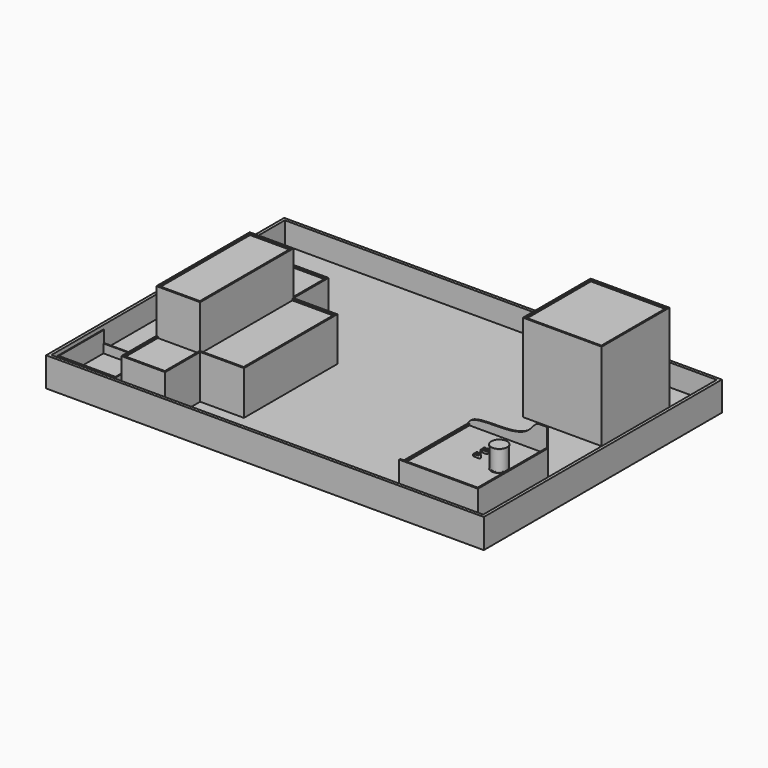
from build123d import *

# Parameters (mm, degrees)
F0_R      = 27.2
F1_DEPTH  = 2.83
F2_R      = 26.4
F3_DEPTH  = 67.36
F4_R      = 27.2
F5_DEPTH  = 2.83
F9_W      = 270
F9_H      = 300
F10_DEPTH = 72
F12_DEPTH = 15
F14_DEPTH = 5
F15_W     = 5
F15_H     = 290
F16_DEPTH = 5
F17_W     = 1500
F17_H     = 1020
F18_DEPTH = 25
F19_W     = 270
F19_H     = 290
F20_DEPTH = 300
F21_W     = 260
F21_H     = 280
F22_DEPTH = 5
F23_W     = 1500
F23_H     = 1020
F23_W_2   = 1480
F23_H_2   = 1000
F24_DEPTH = 75
F26_DEPTH = 150
F27_W     = 150
F27_H     = 400
F28_DEPTH = 150
F29_W     = 140
F29_H     = 390
F30_DEPTH = 5
F31_W     = 140
F31_H     = 145
F31_W_2   = 145
F31_H_2   = 390
F32_DEPTH = 5
F33_R     = 3
F34_DEPTH = 4
F35_R     = 3.99999
F35_2_R   = 3.99999
F36_R     = 3
F37_DEPTH = 8
F38_R     = 3
F39_DEPTH = 8
F40_R     = 3
F40_R_2   = 2.5
F41_DEPTH = 3
F42_R     = 3
F42_R_2   = 2.5
F43_DEPTH = 3
F45_DEPTH = 270.001
F46_W     = 200
F46_H     = 200
F46_W_2   = 194
F46_H_2   = 191
F47_DEPTH = 30
F49_DEPTH = 40
F50_R     = 2.5403619878
F51_DEPTH = 6
F50_R_2   = 2.6285420135
F50_R_3   = 2.461967709
F50_R_4   = 2.4586880428


# Not quite as in the source:
# - a fillet or chamfer is up to 0.001 mm smaller than in the source, because OpenCascade refuses the exact size
# - a feature names something its author has since deleted; it is built from what else it names


with BuildPart() as f1:
    # F0 (on Top) → F1 (new body)
    with BuildSketch(Plane.XY):
        Circle(F0_R)
    extrude(amount=F1_DEPTH)

    # F2 (on face) → F3 (join)
    with BuildSketch(Plane.XY.offset(2.83)):
        Circle(F2_R)
    extrude(amount=F3_DEPTH)

    # F4 (on face) → F5 (join)
    with BuildSketch(Plane.XY.offset(70.19)):
        Circle(F4_R)
    extrude(amount=F5_DEPTH)


with BuildPart() as f10:
    # F9 (on Top) → F10 (new body)
    with BuildSketch(Plane.XY):
        with Locations((-87.8, 0)):
            Rectangle(F9_W, F9_H)
    extrude(amount=-F10_DEPTH)

    # F11 (on face) → F12 (join)
    with BuildSketch(Plane.XY):
        Polygon((-222.8, -145), (-222.8, -150), (47.2, -150), (47.2, 150), (42.2, 150), (42.2, -145), align=None)
    extrude(amount=F12_DEPTH)

    # F13 (on face) → F14 (join)
    with BuildSketch(Plane(origin=(0, 150, 0), x_dir=(-1, 0, 0), z_dir=(0, 1, 0))):
        with BuildLine():
            Line((-21.3134280931, 81.3575685024), (-47.2, 81.3575685024))
            Line((-47.2, 81.3575685024), (-47.2, -72))
            Line((-47.2, -72), (222.8, -72))
            Line((222.8, -72), (222.8, 0))
            add(Edge.make_bspline(
                [(-21.3134280931, 81.3575685024), (-6.3059147253, 81.3822787863), (12.9585432644, 38.1268753575), (103.6097013063, 23.6068887567), (223.0224295336, 30.7718731823), (222.8, 0)],
                knots=[0, 0, 0, 0, 0.2487100673, 0.6151112321, 1, 1, 1, 1], degree=3))
        make_face()
    extrude(amount=-F14_DEPTH)

    # F15 (on face) → F16 (join)
    with BuildSketch(Plane.XY):
        with Locations((-220.3, 0)):
            Rectangle(F15_W, F15_H)
    extrude(amount=F16_DEPTH)

    # F17 (on face) → F18 (join)
    with BuildSketch(Plane(origin=(0, 0, -72), x_dir=(1, 0, 0), z_dir=(0, 0, -1))):
        with Locations((-602.8, -260)):
            Rectangle(F17_W, F17_H)
    extrude(amount=F18_DEPTH)

    # F19 (on face) → F20 (join)
    with BuildSketch(Plane.XY.offset(-72)):
        with Locations((-87.8, 525)):
            Rectangle(F19_W, F19_H)
    extrude(amount=F20_DEPTH)

    # F21 (on face) → F22 (cut)
    with BuildSketch(Plane.XY.offset(228)):
        with Locations((-87.8, 525)):
            Rectangle(F21_W, F21_H)
    extrude(amount=-F22_DEPTH, mode=Mode.SUBTRACT)

    # F23 (on face) → F24 (join)
    with BuildSketch(Plane.XY.offset(-72)):
        with Locations((-602.8, 260)):
            Rectangle(F23_W, F23_H)
        with Locations((-602.8, 260)):
            Rectangle(F23_W_2, F23_H_2, mode=Mode.SUBTRACT)
    extrude(amount=F24_DEPTH)

    # F25 (on face) → F26 (join)
    with BuildSketch(Plane.XY.offset(-72)):
        Polygon((-952.8, 460), (-1102.8, 460), (-1102.8, -240), (-952.8, -240), (-952.8, -90), (-802.8, -90), (-802.8, 310), (-952.8, 310), align=None)
    extrude(amount=F26_DEPTH)

    # F27 (on face) → F28 (join)
    with BuildSketch(Plane.XY.offset(78)):
        with Locations((-1027.8, 110)):
            Rectangle(F27_W, F27_H)
    extrude(amount=F28_DEPTH)

    # F29 (on face) → F30 (cut)
    with BuildSketch(Plane.XY.offset(228)):
        with Locations((-1027.8, 110)):
            Rectangle(F29_W, F29_H)
    extrude(amount=-F30_DEPTH, mode=Mode.SUBTRACT)

    # F31 (on face) → F32 (cut)
    with BuildSketch(Plane.XY.offset(78)):
        with Locations((-1027.8, 382.5)):
            Rectangle(F31_W, F31_H)
        with Locations((-880.3, 110)):
            Rectangle(F31_W_2, F31_H_2)
        with Locations((-1027.8, -162.5)):
            Rectangle(F31_W, F31_H)
    extrude(amount=-F32_DEPTH, mode=Mode.SUBTRACT)

    # F46 (on face) → F47 (join)
    with BuildSketch(Plane.XY.offset(-72)):
        with Locations((-1232.8, -130)):
            Rectangle(F46_W, F46_H)
        with Locations((-1232.8, -128.5)):
            Rectangle(F46_W_2, F46_H_2, mode=Mode.SUBTRACT)
    extrude(amount=F47_DEPTH)

    # F48 (on face) → F49 (join)
    with BuildSketch(Plane.XY.offset(-42)):
        Polygon((-1329.8, -30), (-1332.8, -30), (-1332.8, -230), (-1329.8, -230), (-1135.8, -230), (-1132.8, -230), (-1132.8, -30), (-1135.8, -30), (-1135.8, -224), (-1329.8, -224), align=None)
    extrude(amount=F49_DEPTH)


with BuildPart() as f34:
    # F33 (on offset) → F34 (new body, symmetric)
    with BuildSketch(Plane.XY.offset(25)):
        with BuildLine():
            Line((-55, -12), (-74.5, -12))
            Line((-74.5, -12), (-74.5, -13))
            Line((-74.5, -13), (-65.6457513111, -13))
            ThreePointArc((-65.6457513111, -13), (-67, -16), (-65.6457513111, -19))
            Line((-65.6457513111, -19), (-74.5, -19))
            Line((-74.5, -19), (-74.5, -20))
            Line((-74.5, -20), (-55, -20))
            ThreePointArc((-55, -20), (-51, -16), (-55, -12))
        make_face()
        with Locations((-63, -16)):
            Circle(F33_R, mode=Mode.SUBTRACT)
        with Locations((-55, -16)):
            Circle(F33_R, mode=Mode.SUBTRACT)
    extrude(amount=F34_DEPTH, both=True)

    # F35 (radius 4 in the source; OpenCascade refuses exactly that, so slightly less here)
    f35_edges = [f34.edges().sort_by_distance(p)[0] for p in [
        (-74.5, -19.5, 29),
        (-74.5, -12.5, 29),
        (-74.5, -19.5, 21),
        (-74.5, -12.5, 21),
    ]]
    fillet(f35_edges, radius=F35_R)

    # F36 (on face) → F37 (join, through all)
    with BuildSketch(Plane.XZ.offset(20)):
        with Locations((-70.5, 25)):
            Circle(F36_R)
    extrude(amount=-F37_DEPTH)

    # F42 (on offset) → F43 (join, symmetric)
    with BuildSketch(Plane.XY.offset(25)):
        with Locations((-63, -16)):
            Circle(F42_R)
        with Locations((-63, -16)):
            Circle(F42_R_2, mode=Mode.SUBTRACT)
        with Locations((-55, -16)):
            Circle(F42_R)
        with Locations((-55, -16)):
            Circle(F42_R_2, mode=Mode.SUBTRACT)
    extrude(amount=F43_DEPTH, both=True)


with BuildPart() as f34b:
    # F33 (on offset) → F34, piece 2 (new body, symmetric)
    with BuildSketch(Plane.XY.offset(25)):
        with BuildLine():
            Line((-74.5, 13), (-74.5, 12))
            Line((-74.5, 12), (-55, 12))
            ThreePointArc((-55, 12), (-51, 16), (-55, 20))
            Line((-55, 20), (-74.5, 20))
            Line((-74.5, 20), (-74.5, 19))
            Line((-74.5, 19), (-65.6457513111, 19))
            ThreePointArc((-65.6457513111, 19), (-67, 16), (-65.6457513111, 13))
            Line((-65.6457513111, 13), (-74.5, 13))
        make_face()
        with Locations((-63, 16)):
            Circle(F33_R, mode=Mode.SUBTRACT)
        with Locations((-55, 16)):
            Circle(F33_R, mode=Mode.SUBTRACT)
    extrude(amount=F34_DEPTH, both=True)

    # F35#2 (radius 4 in the source; OpenCascade refuses exactly that, so slightly less here)
    f35_2_edges = [f34b.edges().sort_by_distance(p)[0] for p in [
        (-74.5, 12.5, 29),
        (-74.5, 19.5, 29),
        (-74.5, 19.5, 21),
        (-74.5, 12.5, 21),
    ]]
    fillet(f35_2_edges, radius=F35_2_R)

    # F38 (on face) → F39 (join, through all)
    with BuildSketch(Plane(origin=(0, 20, 0), x_dir=(-1, 0, 0), z_dir=(0, 1, 0))):
        with Locations((70.5, 25)):
            Circle(F38_R)
    extrude(amount=-F39_DEPTH)

    # F40 (on offset) → F41 (join, symmetric)
    with BuildSketch(Plane.XY.offset(25)):
        with Locations((-55, 16)):
            Circle(F40_R)
        with Locations((-55, 16)):
            Circle(F40_R_2, mode=Mode.SUBTRACT)
        with Locations((-63, 16)):
            Circle(F40_R)
        with Locations((-63, 16)):
            Circle(F40_R_2, mode=Mode.SUBTRACT)
    extrude(amount=F41_DEPTH, both=True)


with BuildPart() as f45_tool:
    # F44 (on face) → F45 (new body, through all)
    with BuildSketch(Plane(origin=(0, 20, 0), x_dir=(-1, 0, 0), z_dir=(0, 1, 0))):
        with BuildLine():
            Line((71.5, 26), (71.5, 27.2912878475))
            ThreePointArc((71.5, 27.2912878475), (70.5, 27.5), (69.5, 27.2912878475))
            Line((69.5, 27.2912878475), (69.5, 26))
            Line((69.5, 26), (68.2087121525, 26))
            ThreePointArc((68.2087121525, 26), (68, 25), (68.2087121525, 24))
            Line((68.2087121525, 24), (69.5, 24))
            Line((69.5, 24), (69.5, 22.7087121525))
            ThreePointArc((69.5, 22.7087121525), (70.5, 22.5), (71.5, 22.7087121525))
            Line((71.5, 22.7087121525), (71.5, 24))
            Line((71.5, 24), (72.7912878475, 24))
            ThreePointArc((72.7912878475, 24), (73, 25), (72.7912878475, 26))
            Line((72.7912878475, 26), (71.5, 26))
        make_face()
    extrude(amount=-F45_DEPTH)


with BuildPart() as f34_1:
    add(f34.part)

    # F45: cut by f45_tool
    add(f45_tool.part, mode=Mode.SUBTRACT)


with BuildPart() as f34b_1:
    add(f34b.part)

    # F45: cut by f45_tool
    add(f45_tool.part, mode=Mode.SUBTRACT)


with BuildPart() as f51:
    # F50 (on face) → F51 (new body)
    with BuildSketch(Plane.XY.offset(29)):
        with Locations((-63, 16)):
            Circle(F50_R)
    extrude(amount=F51_DEPTH)


with BuildPart() as f51b:
    # F50 (on face) → F51, piece 2 (new body)
    with BuildSketch(Plane.XY.offset(29)):
        with Locations((-55, 16)):
            Circle(F50_R_2)
    extrude(amount=F51_DEPTH)


with BuildPart() as f51c:
    # F50 (on face) → F51, piece 3 (new body)
    with BuildSketch(Plane.XY.offset(29)):
        with Locations((-55, -15.9977246076)):
            Circle(F50_R_3)
    extrude(amount=F51_DEPTH)


with BuildPart() as f51d:
    # F50 (on face) → F51, piece 4 (new body)
    with BuildSketch(Plane.XY.offset(29)):
        with Locations((-63, -16.0001851618)):
            Circle(F50_R_4)
    extrude(amount=F51_DEPTH)


solid = Compound([f1.part, f10.part, f34_1.part, f34b_1.part, f51.part, f51b.part, f51c.part, f51d.part])
